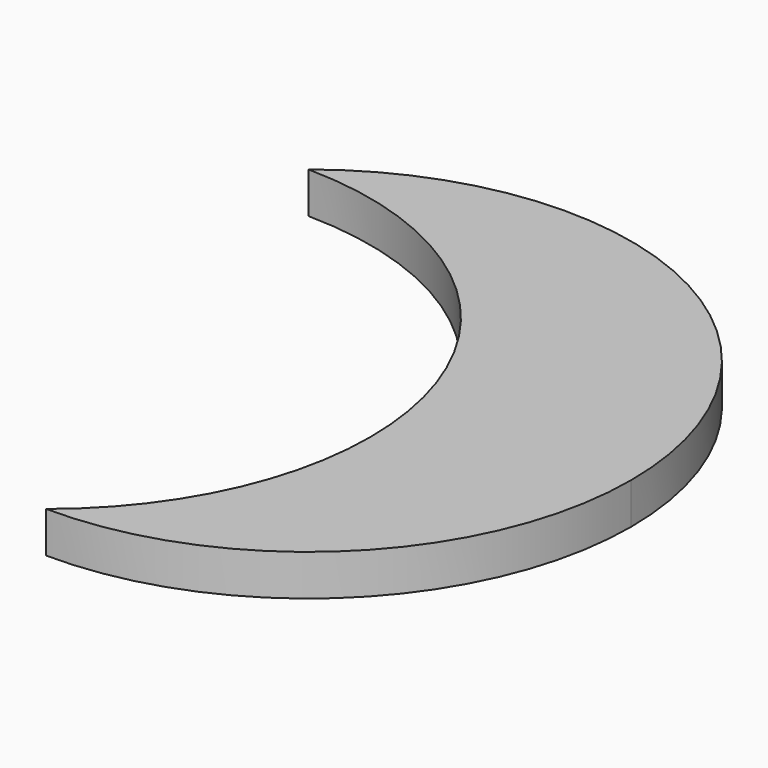
from build123d import *

# Parameters (mm, degrees)
F2_DEPTH = 1.5875


# Not quite as in the source:
# - a length typed as a fraction of an inch, garbled in the dataset ("3 / 203.2 mm" for 3/8 in), is restored


with BuildPart() as f2:
    # F1 (on face) → F2 (new body)
    with BuildSketch(Plane.XY):
        with BuildLine():
            ThreePointArc((168.886805439, -2.726495266), (167.6486102586, -8.1510341004), (164.1792944273, -12.5010451962))
            ThreePointArc((164.1792944273, -12.5010451962), (173.0926609381, -8.8800573298), (176.794584425, 0))
            ThreePointArc((176.794584425, 0), (169.7175607594, 11.2633673196), (156.4989704367, 9.7745499302))
            ThreePointArc((156.4989704367, 9.7745499302), (165.2653002688, 6.0731437471), (168.886805439, -2.726495266))
        make_face()
    extrude(amount=F2_DEPTH)


solid = f2.part
